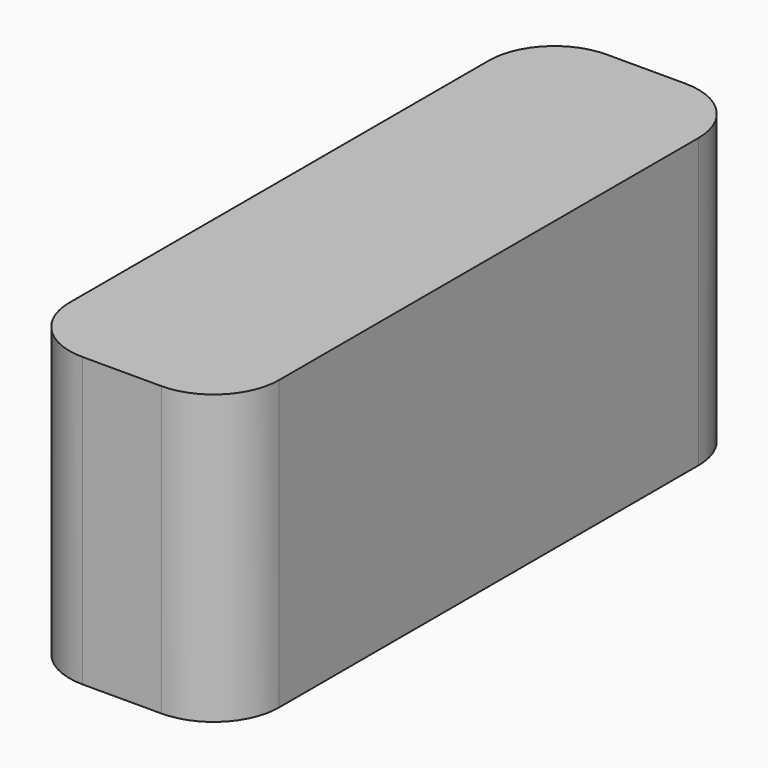
from build123d import *

# Parameters (mm, degrees)
F0_W     = 16
F0_H     = 50
F0_W_2   = 6
F0_H_2   = 40
F1_DEPTH = 12
F2_W     = 16
F2_H     = 50
F3_DEPTH = 10
F4_R     = 4.99999
F5_R     = 5


# Not quite as in the source:
# - a fillet or chamfer is up to 0.001 mm smaller than in the source, because OpenCascade refuses the exact size


with BuildPart() as f1:
    # F0 (on Top) → F1 (new body)
    with BuildSketch(Plane.XY):
        with Locations((-23.0457014143, -5.7597834617)):
            Rectangle(F0_W, F0_H)
        with Locations((-23.0457014143, -5.7597834617)):
            Rectangle(F0_W_2, F0_H_2, mode=Mode.SUBTRACT)
    extrude(amount=F1_DEPTH)

    # F2 (on face) → F3 (join)
    with BuildSketch(Plane.XY.offset(12)):
        with Locations((-23.0457014143, -5.7597834617)):
            Rectangle(F2_W, F2_H)
    extrude(amount=F3_DEPTH)

    # F4 (radius 5 in the source; OpenCascade refuses exactly that, so slightly less here)
    f4_edges = [f1.edges().sort_by_distance(p)[0] for p in [
        (-23.045701, -25.759783, 0),
    ]]
    fillet(f4_edges, radius=F4_R)

    # F5
    f5_edges = [f1.edges().sort_by_distance(p)[0] for p in [
        (-15.045701, 19.240217, 11),
        (-15.045701, -30.759783, 11),
        (-31.045701, -30.759783, 11),
        (-31.045701, 19.240217, 11),
    ]]
    fillet(f5_edges, radius=F5_R)


solid = f1.part
